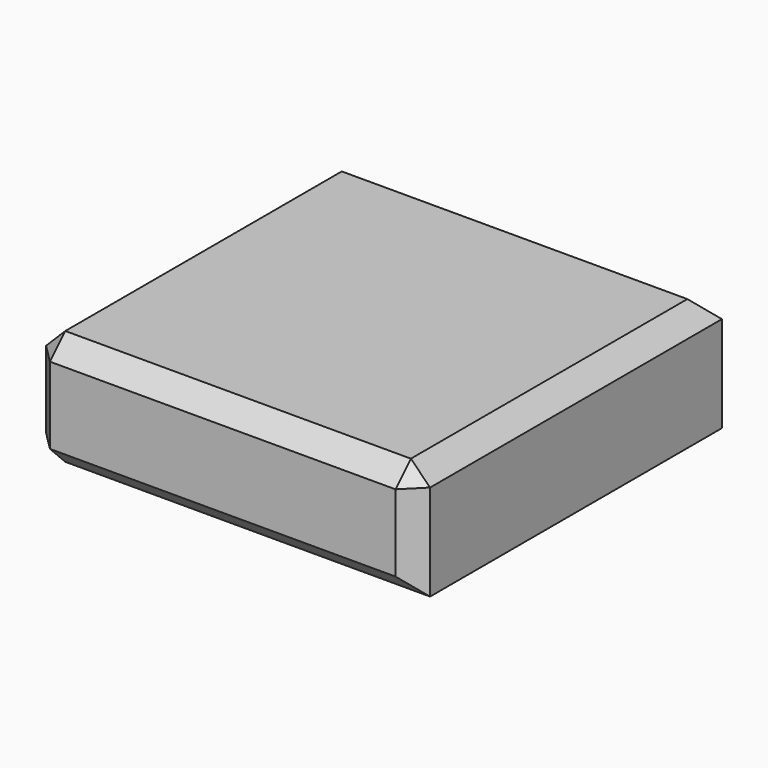
from build123d import *

# Parameters (mm, degrees)
F0_W     = 100
F0_H     = 100
F1_DEPTH = 30
F4_SIZE  = 5


# Not quite as in the source:
# - the program builds the solid bodies; features that only make, move or delete a surface that nothing else refers to are left out


with BuildPart() as f1:
    # F0 (on Top) → F1 (new body)
    with BuildSketch(Plane.XY):
        with Locations((15.8379010856, 10.1181242615)):
            Rectangle(F0_W, F0_H)
    extrude(amount=F1_DEPTH)

    # F4
    f4_edges = [f1.edges().sort_by_distance(p)[0] for p in [
        (65.837901, 10.118124, 30),
        (15.837901, 60.118124, 30),
        (-34.162099, 10.118124, 30),
        (15.837901, -39.881876, 30),
        (-34.162099, -39.881876, 15),
        (65.837901, -39.881876, 15),
        (15.837901, -39.881876, 0),
        (-34.162099, 60.118124, 15),
        (-34.162099, 10.118124, 0),
    ]]
    chamfer(f4_edges, length=F4_SIZE)


solid = f1.part
